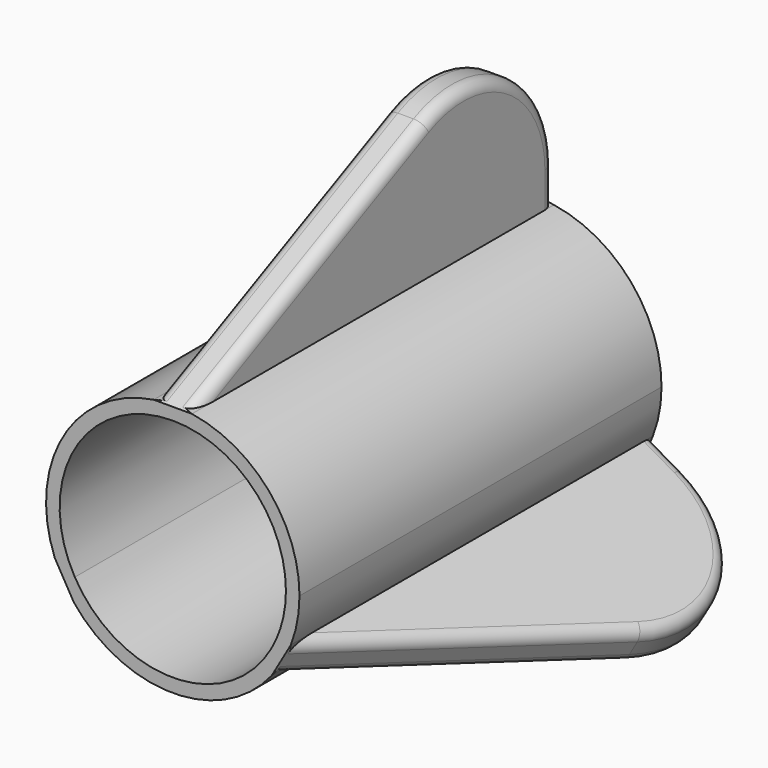
from build123d import *

# Parameters (mm, degrees)
F1_DEPTH      = 20
F2_DEPTH      = 20
F4_DEPTH      = 14.8
F5_R          = 5
F6_DEPTH      = 20
F8_DEPTH      = 25
F10_DEPTH     = 25
F11_R         = 5
F12_T4_DEPTH  = 15.4786422769
F12_S5_R      = 5.6
F12_T6_DEPTH  = 9
F12_T10_DEPTH = 15.4786422769
F12_S11_R     = 5.6
F12_T12_DEPTH = 9
F12_T14_ANGLE = 115.3240588084
F12_T16_ANGLE = 115.3240588084
F12_T20_DEPTH = 2.8166081333
F12_S21_R     = 5.6
F12_T22_DEPTH = 3
F12_T26_DEPTH = 2.8166081333
F12_S27_R     = 5.6
F12_T28_DEPTH = 3
F13_T4_DEPTH  = 15.4786422769
F13_S5_R      = 5.6
F13_T6_DEPTH  = 9
F13_T10_DEPTH = 15.4786422769
F13_S11_R     = 5.6
F13_T12_DEPTH = 10
F13_T16_DEPTH = 15.4786422769
F13_S17_R     = 5.6
F13_T18_DEPTH = 10
F13_T22_DEPTH = 15.4786422769
F13_S23_R     = 5.6
F13_T24_DEPTH = 9
F13_T28_DEPTH = 2.8166081333
F13_S29_R     = 5.6
F13_T30_DEPTH = 3
F13_T34_DEPTH = 2.8166081333
F13_S35_R     = 5.6
F13_T36_DEPTH = 3
F13_T40_DEPTH = 2.8166081333
F13_S41_R     = 5.6
F13_T42_DEPTH = 3
F13_T46_DEPTH = 2.8166081333
F13_S47_R     = 5.6
F13_T48_DEPTH = 3
F13_T50_ANGLE = 115.3240588084
F13_T52_ANGLE = 115.3240588084
F13_T54_ANGLE = 115.3240588084
F13_T56_ANGLE = 115.3240588084


# Not quite as in the source:
# - a fillet or chamfer that OpenCascade refuses, or shapes differently, is made with other operations: its cross-section is extruded or revolved along the edge and cut away or added


with BuildPart() as f1:
    # F0 (on Front) → F1 (new body)
    with BuildSketch(Plane.XZ):
        with BuildLine():
            ThreePointArc((-4.3301270189, -2.5), (-4.3301270189, 2.5), (0, 5))
            Line((0, 5), (-0.8457466924, 5))
            Line((-0.8457466924, 5), (-0.8457466924, 5.5357666617))
            ThreePointArc((-0.8457466924, 5.5357666617), (-4.8497422612, 2.8), (-5.2169879046, -2.03544521))
            Line((-5.2169879046, -2.03544521), (-4.7530003651, -1.7675618792))
            Line((-4.7530003651, -1.7675618792), (-4.3301270189, -2.5))
        make_face()
        with BuildLine():
            Line((3.9072536727, -3.2324381208), (4.3301270189, -2.5))
            ThreePointArc((4.3301270189, -2.5), (0, -5), (-4.3301270189, -2.5))
            Line((-4.3301270189, -2.5), (-3.9072536727, -3.2324381208))
            Line((-3.9072536727, -3.2324381208), (-4.3712412122, -3.5003214516))
            ThreePointArc((-4.3712412122, -3.5003214516), (0, -5.6), (4.3712412122, -3.5003214516))
            Line((4.3712412122, -3.5003214516), (3.9072536727, -3.2324381208))
        make_face()
        with BuildLine():
            Line((-3.9072536727, -3.2324381208), (-4.3301270189, -2.5))
            Line((-4.3301270189, -2.5), (-4.8497422612, -2.8))
            ThreePointArc((-4.8497422612, -2.8), (-4.6237697378, -3.1592330417), (-4.3712412122, -3.5003214516))
            Line((-4.3712412122, -3.5003214516), (-3.9072536727, -3.2324381208))
        make_face()
        with BuildLine():
            Line((-4.8497422612, -2.8), (-4.3301270189, -2.5))
            Line((-4.3301270189, -2.5), (-4.7530003651, -1.7675618792))
            Line((-4.7530003651, -1.7675618792), (-5.2169879046, -2.03544521))
            ThreePointArc((-5.2169879046, -2.03544521), (-5.0478609395, -2.4246855333), (-4.8497422612, -2.8))
        make_face()
        with BuildLine():
            Line((4.8497422612, -2.8), (4.3301270189, -2.5))
            Line((4.3301270189, -2.5), (3.9072536727, -3.2324381208))
            Line((3.9072536727, -3.2324381208), (4.3712412122, -3.5003214516))
            ThreePointArc((4.3712412122, -3.5003214516), (4.6237697378, -3.1592330417), (4.8497422612, -2.8))
        make_face()
        with BuildLine():
            Line((4.7530003651, -1.7675618792), (4.3301270189, -2.5))
            Line((4.3301270189, -2.5), (4.8497422612, -2.8))
            ThreePointArc((4.8497422612, -2.8), (5.0478609395, -2.4246855333), (5.2169879046, -2.03544521))
            Line((5.2169879046, -2.03544521), (4.7530003651, -1.7675618792))
        make_face()
        with BuildLine():
            ThreePointArc((0, 5), (3.5355339059, 3.5355339059), (5, 0))
            ThreePointArc((5, 0), (4.8296291314, -1.2940952255), (4.3301270189, -2.5))
            Line((4.3301270189, -2.5), (4.7530003651, -1.7675618792))
            Line((4.7530003651, -1.7675618792), (5.2169879046, -2.03544521))
            ThreePointArc((5.2169879046, -2.03544521), (5.5034140434, -1.0355838291), (5.6, 0))
            ThreePointArc((5.6, 0), (4.2483044546, 3.6485489254), (0.8457466924, 5.5357666617))
            Line((0.8457466924, 5.5357666617), (0.8457466924, 5))
            Line((0.8457466924, 5), (0, 5))
        make_face()
        with BuildLine():
            Line((0, 5.6), (0, 5))
            Line((0, 5), (0.8457466924, 5))
            Line((0.8457466924, 5), (0.8457466924, 5.5357666617))
            ThreePointArc((0.8457466924, 5.5357666617), (0.4240912017, 5.583918575), (0, 5.6))
        make_face()
        with BuildLine():
            Line((-0.8457466924, 5), (0, 5))
            Line((0, 5), (0, 5.6))
            ThreePointArc((0, 5.6), (-0.4240912017, 5.583918575), (-0.8457466924, 5.5357666617))
            Line((-0.8457466924, 5.5357666617), (-0.8457466924, 5))
        make_face()
    extrude(amount=F1_DEPTH)

    # F0 (on Front) → F2 (join)
    with BuildSketch(Plane.XZ):
        with BuildLine():
            ThreePointArc((-4.3712412122, -3.5003214516), (-4.6237697378, -3.1592330417), (-4.8497422612, -2.8))
            Line((-4.8497422612, -2.8), (-12.9903810568, -7.5))
            Line((-12.9903810568, -7.5), (-12.5675077106, -8.2324381208))
            Line((-12.5675077106, -8.2324381208), (-4.3712412122, -3.5003214516))
        make_face()
        with BuildLine():
            Line((-12.9903810568, -7.5), (-4.8497422612, -2.8))
            ThreePointArc((-4.8497422612, -2.8), (-5.0478609395, -2.4246855333), (-5.2169879046, -2.03544521))
            Line((-5.2169879046, -2.03544521), (-13.413254403, -6.7675618792))
            Line((-13.413254403, -6.7675618792), (-12.9903810568, -7.5))
        make_face()
    extrude(amount=F2_DEPTH)

    # F3 (on face) → F4 (cut)
    with BuildSketch(Plane(origin=(0.4228733462, 0, -0.7324381208), x_dir=(0.8660254038, 0, 0.5), z_dir=(0.5, 0, -0.8660254038))):
        Polygon((-15, 0), (-5.5357666617, 20), (-15, 20), align=None)
    extrude(amount=-F4_DEPTH, mode=Mode.SUBTRACT)

    # F5
    f5_edges = [f1.edges().sort_by_distance(p)[0] for p in [
        (-12.990381, 0, -7.5),
    ]]
    fillet(f5_edges, radius=F5_R)

    # F0 (on Front) → F6 (join)
    with BuildSketch(Plane.XZ):
        with BuildLine():
            ThreePointArc((-0.8457466924, 5.5357666617), (-0.4240912017, 5.583918575), (0, 5.6))
            Line((0, 5.6), (0, 15))
            Line((0, 15), (-0.8457466924, 15))
            Line((-0.8457466924, 15), (-0.8457466924, 5.5357666617))
        make_face()
        with BuildLine():
            Line((0, 15), (0, 5.6))
            ThreePointArc((0, 5.6), (0.4240912017, 5.583918575), (0.8457466924, 5.5357666617))
            Line((0.8457466924, 5.5357666617), (0.8457466924, 15))
            Line((0.8457466924, 15), (0, 15))
        make_face()
        with BuildLine():
            ThreePointArc((5.2169879046, -2.03544521), (5.0478609395, -2.4246855333), (4.8497422612, -2.8))
            Line((4.8497422612, -2.8), (12.9903810568, -7.5))
            Line((12.9903810568, -7.5), (13.413254403, -6.7675618792))
            Line((13.413254403, -6.7675618792), (5.2169879046, -2.03544521))
        make_face()
        with BuildLine():
            Line((12.9903810568, -7.5), (4.8497422612, -2.8))
            ThreePointArc((4.8497422612, -2.8), (4.6237697378, -3.1592330417), (4.3712412122, -3.5003214516))
            Line((4.3712412122, -3.5003214516), (12.5675077106, -8.2324381208))
            Line((12.5675077106, -8.2324381208), (12.9903810568, -7.5))
        make_face()
    extrude(amount=F6_DEPTH)

    # F7 (on face) → F8 (cut)
    with BuildSketch(Plane(origin=(0.4228733462, 0, 0.7324381208), x_dir=(0.8660254038, 0, -0.5), z_dir=(0.5, 0, 0.8660254038))):
        Polygon((15, 0), (5.5357666617, -20), (15, -20), align=None)
    extrude(amount=-F8_DEPTH, mode=Mode.SUBTRACT)

    # F9 (on face) → F10 (cut)
    with BuildSketch(Plane.YZ.offset(0.8457466924)):
        Polygon((-20, 15), (-20, 5.5357666617), (0, 15), align=None)
    extrude(amount=-F10_DEPTH, mode=Mode.SUBTRACT)

    # F11
    f11_edges = [f1.edges().sort_by_distance(p)[0] for p in [
        (12.990381, 0, -7.5),
        (0, 0, 15),
    ]]
    fillet(f11_edges, radius=F11_R)

    # F12: fillet of radius 0.5 on 4 edges, made by hand


with BuildPart() as f12_tool2:
    # F12_s3 → F12_t4 (new body)
    with BuildSketch(Plane(origin=(0, -15.3303811163, -7.2545152025), x_dir=(1, 0, 0), z_dir=(0, 0.9039030201, 0.4277374549))):
        with BuildLine():
            ThreePointArc((0.8457466924, -13.0585453012), (0.699300083, -13.4120986918), (0.3457466924, -13.5585453012))
            Line((0.3457466924, -13.5585453012), (0.8457466924, -13.5585453012))
            Line((0.8457466924, -13.5585453012), (0.8457466924, -13.0585453012))
        make_face()
    extrude(amount=F12_T4_DEPTH)

    # F12_s5 → F12_t6 (cut, symmetric)
    with BuildSketch(Plane.XZ.offset(14)):
        Circle(F12_S5_R)
    extrude(amount=F12_T6_DEPTH, both=True, mode=Mode.SUBTRACT)


with BuildPart() as f1_1:
    add(f1.part)

    # F12_t1: cut F12_tool2
    add(f12_tool2.part, mode=Mode.SUBTRACT)


with BuildPart() as f12_tool8:
    # F12_s9 → F12_t10 (new body)
    with BuildSketch(Plane(origin=(0, -15.3303811163, -7.2545152025), x_dir=(1, 0, 0), z_dir=(0, 0.9039030201, 0.4277374549))):
        with BuildLine():
            ThreePointArc((-0.8457466924, -13.0585453012), (-0.699300083, -13.4120986918), (-0.3457466924, -13.5585453012))
            Line((-0.3457466924, -13.5585453012), (-0.8457466924, -13.5585453012))
            Line((-0.8457466924, -13.5585453012), (-0.8457466924, -13.0585453012))
        make_face()
    extrude(amount=F12_T10_DEPTH)

    # F12_s11 → F12_t12 (cut, symmetric)
    with BuildSketch(Plane.XZ.offset(14)):
        Circle(F12_S11_R)
    extrude(amount=F12_T12_DEPTH, both=True, mode=Mode.SUBTRACT)


with BuildPart() as f1_2:
    add(f1_1.part)

    # F12_t7: cut F12_tool8
    add(f12_tool8.part, mode=Mode.SUBTRACT)

    # F12_s13 → F12_t14 (revolve, cut)
    with BuildSketch(Plane.XY.offset(7.1023747949)):
        with BuildLine():
            ThreePointArc((0.8457466924, -0.5), (0.699300083, -0.1464466094), (0.3457466924, 0))
            Line((0.3457466924, 0), (0.8457466924, 0))
            Line((0.8457466924, 0), (0.8457466924, -0.5))
        make_face()
    revolve(axis=Axis((0.8457466924, -5, 7.1023747949), (1, 0, 0)), revolution_arc=F12_T14_ANGLE, mode=Mode.SUBTRACT)

    # F12_s15 → F12_t16 (revolve, cut)
    with BuildSketch(Plane.XY.offset(7.1023747949)):
        with BuildLine():
            ThreePointArc((-0.3457466924, 0), (-0.699300083, -0.1464466094), (-0.8457466924, -0.5))
            Line((-0.8457466924, -0.5), (-0.8457466924, 0))
            Line((-0.8457466924, 0), (-0.3457466924, 0))
        make_face()
    revolve(axis=Axis((-0.8457466924, -5, 7.1023747949), (1, 0, 0)), revolution_arc=F12_T16_ANGLE, mode=Mode.SUBTRACT)


with BuildPart() as f12_tool18:
    # F12_s19 → F12_t20 (new body)
    with BuildSketch(Plane.XY.offset(7.1023747949)):
        with BuildLine():
            ThreePointArc((-0.3457466924, 0), (-0.699300083, -0.1464466094), (-0.8457466924, -0.5))
            Line((-0.8457466924, -0.5), (-0.8457466924, 0))
            Line((-0.8457466924, 0), (-0.3457466924, 0))
        make_face()
    extrude(amount=-F12_T20_DEPTH)

    # F12_s21 → F12_t22 (cut, symmetric)
    with BuildSketch(Plane.XZ.offset(0.2)):
        Circle(F12_S21_R)
    extrude(amount=F12_T22_DEPTH, both=True, mode=Mode.SUBTRACT)


with BuildPart() as f1_3:
    add(f1_2.part)

    # F12_t17: cut F12_tool18
    add(f12_tool18.part, mode=Mode.SUBTRACT)


with BuildPart() as f12_tool24:
    # F12_s25 → F12_t26 (new body)
    with BuildSketch(Plane.XY.offset(4.2857666617)):
        with BuildLine():
            ThreePointArc((0.3457466924, 0), (0.699300083, -0.1464466094), (0.8457466924, -0.5))
            Line((0.8457466924, -0.5), (0.8457466924, 0))
            Line((0.8457466924, 0), (0.3457466924, 0))
        make_face()
    extrude(amount=F12_T26_DEPTH)

    # F12_s27 → F12_t28 (cut, symmetric)
    with BuildSketch(Plane.XZ.offset(0.2)):
        Circle(F12_S27_R)
    extrude(amount=F12_T28_DEPTH, both=True, mode=Mode.SUBTRACT)


with BuildPart() as f1_4:
    add(f1_3.part)

    # F12_t23: cut F12_tool24
    add(f12_tool24.part, mode=Mode.SUBTRACT)

    # F13: fillet of radius 0.5 on 12 edges, made by hand


with BuildPart() as f13_tool2:
    # F13_s3 → F13_t4 (new body)
    with BuildSketch(Plane(origin=(-0.548817749, -1.3391896155, 0.3168600751), x_dir=(0.9253125221, -0.3792054013, 0), z_dir=(-0.3704315021, -0.9039030201, 0.2138687274))):
        with BuildLine():
            ThreePointArc((11.9681833862, -5.2918313734), (12.2138673733, -5.5852355109), (12.1801241312, -5.9664283795))
            Line((12.1801241312, -5.9664283795), (12.4114522618, -5.5231595039))
            Line((12.4114522618, -5.5231595039), (11.9681833862, -5.2918313734))
        make_face()
    extrude(amount=F13_T4_DEPTH)

    # F13_s5 → F13_t6 (cut, symmetric)
    with BuildSketch(Plane.XZ.offset(14)):
        Circle(F13_S5_R)
    extrude(amount=F13_T6_DEPTH, both=True, mode=Mode.SUBTRACT)


with BuildPart() as f1_5:
    add(f1_4.part)

    # F13_t1: cut F13_tool2
    add(f13_tool2.part, mode=Mode.SUBTRACT)


with BuildPart() as f13_tool8:
    # F13_s9 → F13_t10 (new body)
    with BuildSketch(Plane(origin=(-0.548817749, -1.3391896155, 0.3168600751), x_dir=(0.9253125221, -0.3792054013, 0), z_dir=(-0.3704315021, -0.9039030201, 0.2138687274))):
        with BuildLine():
            ThreePointArc((11.1856033812, -6.7914041148), (11.5667962497, -6.8251473568), (11.8602003872, -6.5794633698))
            Line((11.8602003872, -6.5794633698), (11.6288722567, -7.0227322453))
            Line((11.6288722567, -7.0227322453), (11.1856033812, -6.7914041148))
        make_face()
    extrude(amount=F13_T10_DEPTH)

    # F13_s11 → F13_t12 (cut, symmetric)
    with BuildSketch(Plane.XZ.offset(14)):
        Circle(F13_S11_R)
    extrude(amount=F13_T12_DEPTH, both=True, mode=Mode.SUBTRACT)


with BuildPart() as f1_6:
    add(f1_5.part)

    # F13_t7: cut F13_tool8
    add(f13_tool8.part, mode=Mode.SUBTRACT)


with BuildPart() as f13_tool14:
    # F13_s15 → F13_t16 (new body)
    with BuildSketch(Plane(origin=(0.548817749, -1.3391896155, 0.3168600751), x_dir=(0.9253125221, 0.3792054013, 0), z_dir=(0.3704315021, -0.9039030201, 0.2138687274))):
        with BuildLine():
            ThreePointArc((-11.1856033812, -6.7914041148), (-11.5667962497, -6.8251473568), (-11.8602003872, -6.5794633698))
            Line((-11.8602003872, -6.5794633698), (-11.6288722567, -7.0227322453))
            Line((-11.6288722567, -7.0227322453), (-11.1856033812, -6.7914041148))
        make_face()
    extrude(amount=F13_T16_DEPTH)

    # F13_s17 → F13_t18 (cut, symmetric)
    with BuildSketch(Plane.XZ.offset(14)):
        Circle(F13_S17_R)
    extrude(amount=F13_T18_DEPTH, both=True, mode=Mode.SUBTRACT)


with BuildPart() as f1_7:
    add(f1_6.part)

    # F13_t13: cut F13_tool14
    add(f13_tool14.part, mode=Mode.SUBTRACT)


with BuildPart() as f13_tool20:
    # F13_s21 → F13_t22 (new body)
    with BuildSketch(Plane(origin=(0.548817749, -1.3391896155, 0.3168600751), x_dir=(0.9253125221, 0.3792054013, 0), z_dir=(0.3704315021, -0.9039030201, 0.2138687274))):
        with BuildLine():
            ThreePointArc((-11.9681833862, -5.2918313734), (-12.2138673733, -5.5852355109), (-12.1801241312, -5.9664283795))
            Line((-12.1801241312, -5.9664283795), (-12.4114522618, -5.5231595039))
            Line((-12.4114522618, -5.5231595039), (-11.9681833862, -5.2918313734))
        make_face()
    extrude(amount=F13_T22_DEPTH)

    # F13_s23 → F13_t24 (cut, symmetric)
    with BuildSketch(Plane.XZ.offset(14)):
        Circle(F13_S23_R)
    extrude(amount=F13_T24_DEPTH, both=True, mode=Mode.SUBTRACT)


with BuildPart() as f1_8:
    add(f1_7.part)

    # F13_t19: cut F13_tool20
    add(f13_tool20.part, mode=Mode.SUBTRACT)


with BuildPart() as f13_tool26:
    # F13_s27 → F13_t28 (new body)
    with BuildSketch(Plane(origin=(3.7115828037, 0, -2.1428833308), x_dir=(0, 1, 0), z_dir=(0.8660254038, 0, -0.5))):
        with BuildLine():
            ThreePointArc((0, -0.3457466924), (-0.1464466094, -0.699300083), (-0.5, -0.8457466924))
            Line((-0.5, -0.8457466924), (0, -0.8457466924))
            Line((0, -0.8457466924), (0, -0.3457466924))
        make_face()
    extrude(amount=F13_T28_DEPTH)

    # F13_s29 → F13_t30 (cut, symmetric)
    with BuildSketch(Plane.XZ.offset(0.2)):
        Circle(F13_S29_R)
    extrude(amount=F13_T30_DEPTH, both=True, mode=Mode.SUBTRACT)


with BuildPart() as f1_9:
    add(f1_8.part)

    # F13_t25: cut F13_tool26
    add(f13_tool26.part, mode=Mode.SUBTRACT)


with BuildPart() as f13_tool32:
    # F13_s33 → F13_t34 (new body)
    with BuildSketch(Plane(origin=(-6.1508369996, 0, -3.5511873975), x_dir=(0, 1, 0), z_dir=(0.8660254038, 0, 0.5))):
        with BuildLine():
            ThreePointArc((0, -0.3457466924), (-0.1464466094, -0.699300083), (-0.5, -0.8457466924))
            Line((-0.5, -0.8457466924), (0, -0.8457466924))
            Line((0, -0.8457466924), (0, -0.3457466924))
        make_face()
    extrude(amount=F13_T34_DEPTH)

    # F13_s35 → F13_t36 (cut, symmetric)
    with BuildSketch(Plane.XZ.offset(0.3)):
        Circle(F13_S35_R)
    extrude(amount=F13_T36_DEPTH, both=True, mode=Mode.SUBTRACT)


with BuildPart() as f1_10:
    add(f1_9.part)

    # F13_t31: cut F13_tool32
    add(f13_tool32.part, mode=Mode.SUBTRACT)


with BuildPart() as f13_tool38:
    # F13_s39 → F13_t40 (new body)
    with BuildSketch(Plane(origin=(-3.7115828037, 0, -2.1428833308), x_dir=(0, 1, 0), z_dir=(-0.8660254038, 0, -0.5))):
        with BuildLine():
            ThreePointArc((0, -0.3457466924), (-0.1464466094, -0.699300083), (-0.5, -0.8457466924))
            Line((-0.5, -0.8457466924), (0, -0.8457466924))
            Line((0, -0.8457466924), (0, -0.3457466924))
        make_face()
    extrude(amount=F13_T40_DEPTH)

    # F13_s41 → F13_t42 (cut, symmetric)
    with BuildSketch(Plane.XZ.offset(0.3)):
        Circle(F13_S41_R)
    extrude(amount=F13_T42_DEPTH, both=True, mode=Mode.SUBTRACT)


with BuildPart() as f1_11:
    add(f1_10.part)

    # F13_t37: cut F13_tool38
    add(f13_tool38.part, mode=Mode.SUBTRACT)


with BuildPart() as f13_tool44:
    # F13_s45 → F13_t46 (new body)
    with BuildSketch(Plane(origin=(6.1508369996, 0, -3.5511873975), x_dir=(0, 1, 0), z_dir=(-0.8660254038, 0, 0.5))):
        with BuildLine():
            ThreePointArc((0, -0.3457466924), (-0.1464466094, -0.699300083), (-0.5, -0.8457466924))
            Line((-0.5, -0.8457466924), (0, -0.8457466924))
            Line((0, -0.8457466924), (0, -0.3457466924))
        make_face()
    extrude(amount=F13_T46_DEPTH)

    # F13_s47 → F13_t48 (cut, symmetric)
    with BuildSketch(Plane.XZ.offset(0.2)):
        Circle(F13_S47_R)
    extrude(amount=F13_T48_DEPTH, both=True, mode=Mode.SUBTRACT)


with BuildPart() as f1_12:
    add(f1_11.part)

    # F13_t43: cut F13_tool44
    add(f13_tool44.part, mode=Mode.SUBTRACT)

    # F13_s49 → F13_t50 (revolve, cut)
    with BuildSketch(Plane(origin=(6.1508369996, 0, -3.5511873975), x_dir=(0, 1, 0), z_dir=(-0.8660254038, 0, 0.5))):
        with BuildLine():
            ThreePointArc((-0.5, 0.8457466924), (-0.1464466094, 0.699300083), (0, 0.3457466924))
            Line((0, 0.3457466924), (0, 0.8457466924))
            Line((0, 0.8457466924), (-0.5, 0.8457466924))
        make_face()
    revolve(axis=Axis((5.7279636534, -5, -4.2836255183), (-0.5, 0, -0.8660254038)), revolution_arc=F13_T50_ANGLE, mode=Mode.SUBTRACT)

    # F13_s51 → F13_t52 (revolve, cut)
    with BuildSketch(Plane(origin=(-6.1508369996, 0, -3.5511873975), x_dir=(0, 1, 0), z_dir=(0.8660254038, 0, 0.5))):
        with BuildLine():
            ThreePointArc((-0.5, -0.8457466924), (-0.1464466094, -0.699300083), (0, -0.3457466924))
            Line((0, -0.3457466924), (0, -0.8457466924))
            Line((0, -0.8457466924), (-0.5, -0.8457466924))
        make_face()
    revolve(axis=Axis((-5.7279636534, -5, -4.2836255183), (-0.5, 0, 0.8660254038)), revolution_arc=F13_T52_ANGLE, mode=Mode.SUBTRACT)

    # F13_s53 → F13_t54 (revolve, cut)
    with BuildSketch(Plane(origin=(-6.1508369996, 0, -3.5511873975), x_dir=(0, 1, 0), z_dir=(0.8660254038, 0, 0.5))):
        with BuildLine():
            ThreePointArc((0, 0.3457466924), (-0.1464466094, 0.699300083), (-0.5, 0.8457466924))
            Line((-0.5, 0.8457466924), (0, 0.8457466924))
            Line((0, 0.8457466924), (0, 0.3457466924))
        make_face()
    revolve(axis=Axis((-6.5737103458, -5, -2.8187492767), (-0.5, 0, 0.8660254038)), revolution_arc=F13_T54_ANGLE, mode=Mode.SUBTRACT)

    # F13_s55 → F13_t56 (revolve, cut)
    with BuildSketch(Plane(origin=(6.1508369996, 0, -3.5511873975), x_dir=(0, 1, 0), z_dir=(-0.8660254038, 0, 0.5))):
        with BuildLine():
            ThreePointArc((-0.5, -0.8457466924), (-0.1464466094, -0.699300083), (0, -0.3457466924))
            Line((0, -0.3457466924), (0, -0.8457466924))
            Line((0, -0.8457466924), (-0.5, -0.8457466924))
        make_face()
    revolve(axis=Axis((6.5737103458, -5, -2.8187492767), (-0.5, 0, -0.8660254038)), revolution_arc=F13_T56_ANGLE, mode=Mode.SUBTRACT)


solid = f1_12.part
